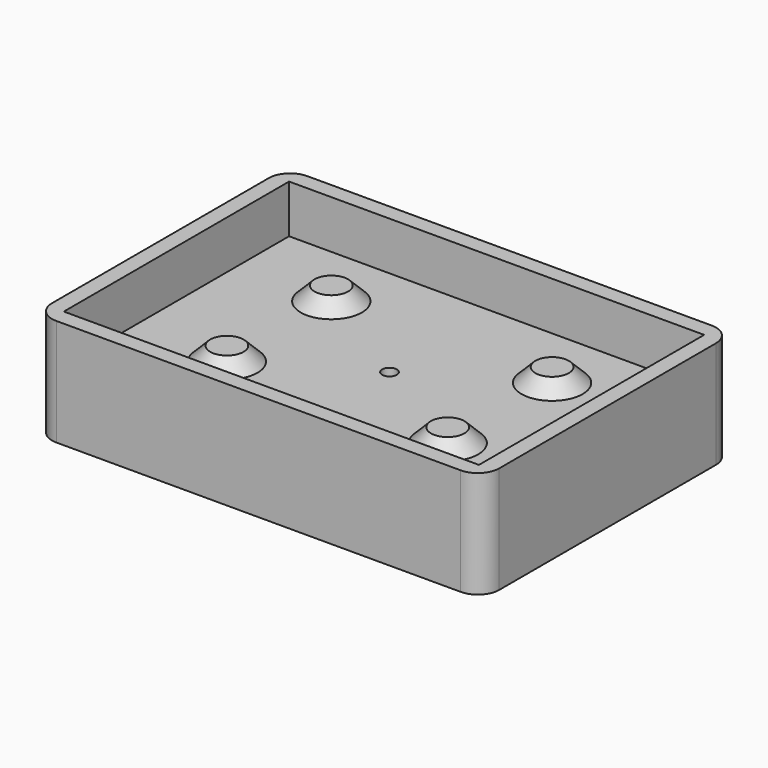
from build123d import *

# Parameters (mm, degrees)
F0_W     = 106.1315912282
F0_H     = 74.4450837374
F0_W_2   = 98.5115912282
F0_H_2   = 66.8250837374
F1_DEPTH = 25.4
F0_R     = 9.0429354427
F2_DEPTH = 13.97
F3_DEPTH = 17.272
F4_D     = 3.5
F6_R     = 5.08


# Not quite as in the source:
# - a fillet or chamfer that OpenCascade refuses, or shapes differently, is made with other operations: its cross-section is extruded or revolved along the edge and cut away or added


with BuildPart() as f1:
    # F0 (on Top) → F1 (new body)
    with BuildSketch(Plane.XY):
        with Locations((0.6595404583, -2.4548470974)):
            Rectangle(F0_W, F0_H)
        with Locations((0.6595404583, -2.4548470974)):
            Rectangle(F0_W_2, F0_H_2, mode=Mode.SUBTRACT)
    extrude(amount=F1_DEPTH)

    # F0 (on Top) → F2 (join)
    with BuildSketch(Plane.XY):
        with Locations((0.6595404583, -2.4548470974)):
            Rectangle(F0_W_2, F0_H_2)
        with Locations((-26.1980332434, -15.4872145504)):
            Circle(F0_R, mode=Mode.SUBTRACT)
        with Locations((26.1980332434, -15.4872145504)):
            Circle(F0_R, mode=Mode.SUBTRACT)
        with Locations((-26.1980332434, 15.4872145504)):
            Circle(F0_R, mode=Mode.SUBTRACT)
        with Locations((26.1980332434, 15.4872145504)):
            Circle(F0_R, mode=Mode.SUBTRACT)
    extrude(amount=F2_DEPTH)

    # F0 (on Top) → F3 (join)
    with BuildSketch(Plane.XY):
        with Locations((-26.1980332434, -15.4872145504)):
            Circle(F0_R)
        with Locations((-26.1980332434, 15.4872145504)):
            Circle(F0_R)
        with Locations((26.1980332434, 15.4872145504)):
            Circle(F0_R)
        with Locations((26.1980332434, -15.4872145504)):
            Circle(F0_R)
    extrude(amount=F3_DEPTH)

    # F4 (through all)
    with Locations(Plane(origin=(0, 0, 0), x_dir=(1, 0, 0), z_dir=(0, 0, -1))):
        with Locations((0, 0)):
            Hole(F4_D / 2)

    # F5: chamfer of 5.08 on 4 edges, made by hand


with BuildPart() as f5_tool2:
    # F5_s3 → F5_t4 (revolve)
    with BuildSketch(Plane.XZ.offset(-15.4872145504)):
        Polygon((-17.1550978007, 12.192), (-22.2350978007, 17.272), (-17.1550978007, 17.272), align=None)
    revolve(axis=Axis((-26.1980332434, 15.4872145504, 17.272), (0, 0, 1)))

    split(bisect_by=Plane.XY.offset(13.97), keep=Keep.TOP)


with BuildPart() as f1_1:
    add(f1.part)

    # F5_t1: cut F5_tool2
    add(f5_tool2.part, mode=Mode.SUBTRACT)


with BuildPart() as f5_tool7:
    # F5_s8 → F5_t9 (revolve)
    with BuildSketch(Plane.XZ.offset(-15.4872145504)):
        Polygon((35.2409686861, 12.192), (30.1609686861, 17.272), (35.2409686861, 17.272), align=None)
    revolve(axis=Axis((26.1980332434, 15.4872145504, 17.272), (0, 0, 1)))

    split(bisect_by=Plane.XY.offset(13.97), keep=Keep.TOP)


with BuildPart() as f1_2:
    add(f1_1.part)

    # F5_t6: cut F5_tool7
    add(f5_tool7.part, mode=Mode.SUBTRACT)


with BuildPart() as f5_tool12:
    # F5_s13 → F5_t14 (revolve)
    with BuildSketch(Plane.XZ.offset(15.4872145504)):
        Polygon((35.2409686861, 12.192), (30.1609686861, 17.272), (35.2409686861, 17.272), align=None)
    revolve(axis=Axis((26.1980332434, -15.4872145504, 17.272), (0, 0, 1)))

    split(bisect_by=Plane.XY.offset(13.97), keep=Keep.TOP)


with BuildPart() as f1_3:
    add(f1_2.part)

    # F5_t11: cut F5_tool12
    add(f5_tool12.part, mode=Mode.SUBTRACT)


with BuildPart() as f5_tool17:
    # F5_s18 → F5_t19 (revolve)
    with BuildSketch(Plane.XZ.offset(15.4872145504)):
        Polygon((-17.1550978007, 12.192), (-22.2350978007, 17.272), (-17.1550978007, 17.272), align=None)
    revolve(axis=Axis((-26.1980332434, -15.4872145504, 17.272), (0, 0, 1)))

    split(bisect_by=Plane.XY.offset(13.97), keep=Keep.TOP)


with BuildPart() as f1_4:
    add(f1_3.part)

    # F5_t16: cut F5_tool17
    add(f5_tool17.part, mode=Mode.SUBTRACT)

    # F6
    f6_edges = [f1_4.edges().sort_by_distance(p)[0] for p in [
        (-52.406255, -39.677389, 12.7),
        (-52.406255, 34.767695, 12.7),
        (53.725336, -39.677389, 12.7),
        (53.725336, 34.767695, 12.7),
    ]]
    fillet(f6_edges, radius=F6_R)


solid = f1_4.part
